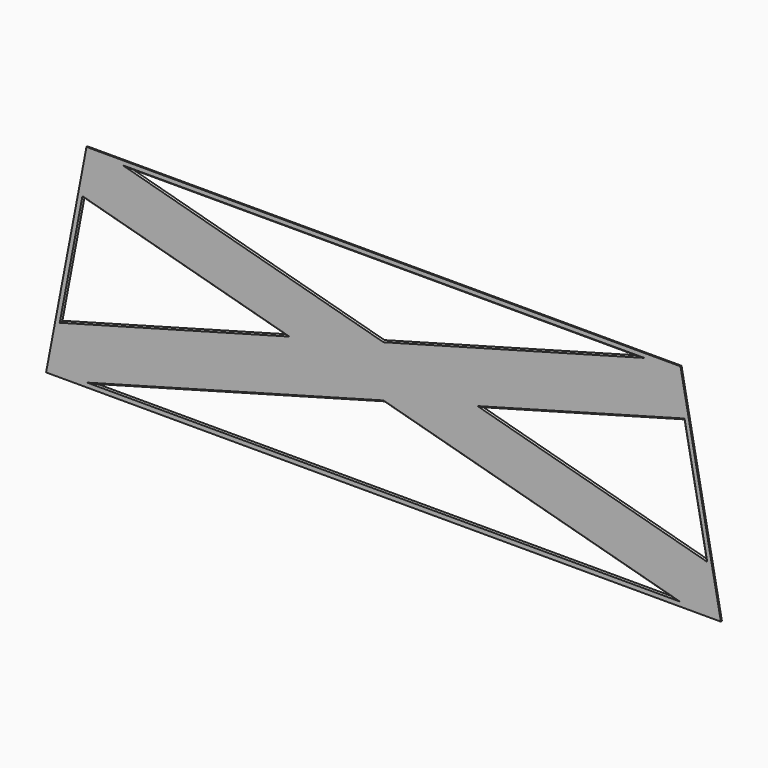
from build123d import *

# Parameters (mm, degrees)
F1_DEPTH = 3.175
F2_SIZE  = 3.17499


# Not quite as in the source:
# - a fillet or chamfer is up to 0.001 mm smaller than in the source, because OpenCascade refuses the exact size


with BuildPart() as f1:
    # F0 (on Front) → F1 (new body)
    with BuildSketch(Plane.XZ):
        Polygon((99.3750451773, 520.7), (0, 0), (1660.017, 0), (1560.6419548227, 520.7), align=None)
        Polygon((1535.1786987879, 13.97), (124.8383012121, 13.97), (830.0085, 205.9645134825), align=None, mode=Mode.SUBTRACT)
        Polygon((37.6746165108, 122.8850133893), (91.8845400349, 406.9312458074), (586.4115107328, 272.2879138766), align=None, mode=Mode.SUBTRACT)
        Polygon((1568.1324599651, 406.9312458074), (1622.3423834892, 122.8850133893), (1073.6054892672, 272.2879138766), align=None, mode=Mode.SUBTRACT)
        Polygon((830.0085, 338.6113142706), (212.5310268921, 506.73), (1447.4859731079, 506.73), align=None, mode=Mode.SUBTRACT)
    extrude(amount=F1_DEPTH)

    # F2 (size 3.175 in the source; OpenCascade refuses exactly that, so slightly less here)
    f2_edges = [f1.edges().sort_by_distance(p)[0] for p in [
        (64.779578, -3.175, 264.90813),
        (312.043064, -3.175, 197.586464),
        (339.148025, -3.175, 339.60958),
        (521.269763, -3.175, 422.670657),
        (830.0085, -3.175, 506.73),
        (1138.747237, -3.175, 422.670657),
        (1320.868975, -3.175, 339.60958),
        (1347.973936, -3.175, 197.586464),
        (1595.237422, -3.175, 264.90813),
        (830.0085, -3.175, 13.97),
        (1182.593599, -3.175, 109.967257),
        (477.423401, -3.175, 109.967257),
    ]]
    chamfer(f2_edges, length=F2_SIZE)


solid = f1.part
